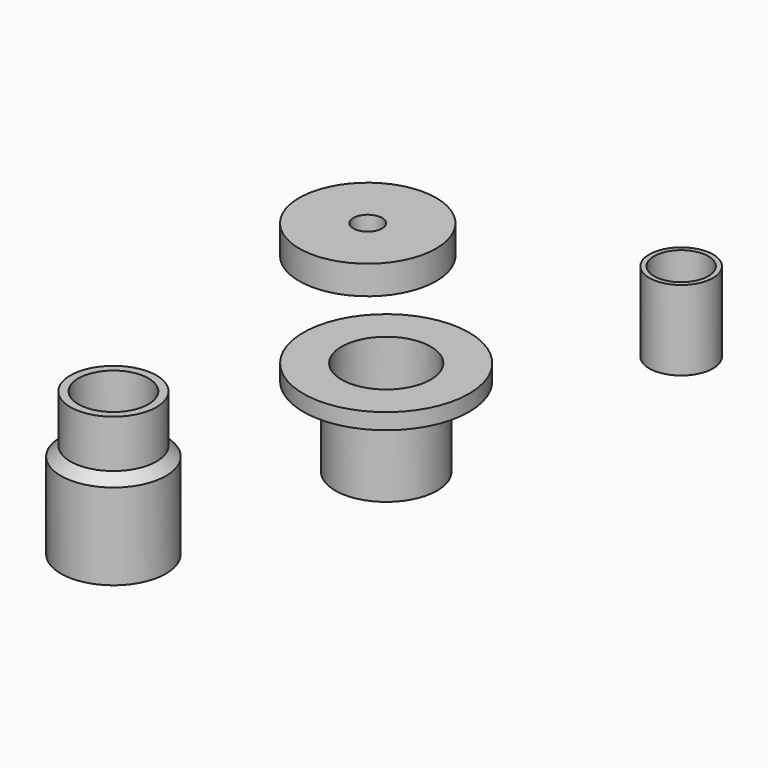
from build123d import *

# Parameters (mm, degrees)
F0_R      = 26
F0_R_2    = 14
F1_DEPTH  = 5
F2_R      = 16
F2_R_2    = 14
F3_DEPTH  = 25
F4_R      = 13.5
F4_R_2    = 11
F5_DEPTH  = 15
F6_R      = 16.5
F7_DEPTH  = 30
F8_SIZE2  = 2.99999
F8_SIZE   = 2.99999
F9_R      = 10
F9_R_2    = 2
F10_DEPTH = 25
F11_R     = 8.5
F12_DEPTH = 15
F13_R     = 3.25
F14_DEPTH = 8
F15_R     = 21.5
F15_R_2   = 4.5
F16_DEPTH = 9


# Not quite as in the source:
# - a fillet or chamfer is up to 0.001 mm smaller than in the source, because OpenCascade refuses the exact size


with BuildPart() as f1:
    # F0 (on Top) → F1 (new body)
    with BuildSketch(Plane.XY):
        Circle(F0_R)
        Circle(F0_R_2, mode=Mode.SUBTRACT)
    extrude(amount=F1_DEPTH)

    # F2 (on face) → F3 (join)
    with BuildSketch(Plane(origin=(0, 0, 0), x_dir=(1, 0, 0), z_dir=(0, 0, -1))):
        Circle(F2_R)
        Circle(F2_R_2, mode=Mode.SUBTRACT)
    extrude(amount=F3_DEPTH)


with BuildPart() as f5:
    # F4 (on Top) → F5 (new body)
    with BuildSketch(Plane.XY):
        with Locations((-48.8465763628, -45.8897389472)):
            Circle(F4_R)
        with Locations((-48.8465763628, -45.8897389472)):
            Circle(F4_R_2, mode=Mode.SUBTRACT)
    extrude(amount=-F5_DEPTH)

    # F6 (on face) → F7 (join)
    with BuildSketch(Plane(origin=(0, 0, -15), x_dir=(1, 0, 0), z_dir=(0, 0, -1))):
        with Locations((-48.8465763628, 45.8897389472)):
            Circle(F6_R)
    extrude(amount=F7_DEPTH)

    # F8 (size 3 and 3 in the source; OpenCascade refuses exactly that, so slightly less here)
    f8_edges = [f5.edges().sort_by_distance(p)[0] for p in [
        (-65.346576, -45.889739, -15),
    ]]
    chamfer(f8_edges, length=F8_SIZE, length2=F8_SIZE2)


with BuildPart() as f10:
    # F9 (on Top) → F10 (new body)
    with BuildSketch(Plane.XY):
        with Locations((48.2846722007, 55.2974492311)):
            Circle(F9_R)
        with Locations((48.2846722007, 55.2974492311)):
            Circle(F9_R_2, mode=Mode.SUBTRACT)
    extrude(amount=F10_DEPTH)

    # F11 (on face) → F12 (cut)
    with BuildSketch(Plane.XY.offset(25)):
        with Locations((48.2846722007, 55.2974492311)):
            Circle(F11_R)
    extrude(amount=-F12_DEPTH, mode=Mode.SUBTRACT)

    # F13 (on face) → F14 (cut)
    with BuildSketch(Plane.XY.offset(10)):
        with Locations((48.2846722007, 55.2974492311)):
            Circle(F13_R)
    extrude(amount=-F14_DEPTH, mode=Mode.SUBTRACT)


with BuildPart() as f16:
    # F15 (on Top) → F16 (new body)
    with BuildSketch(Plane.XY):
        with Locations((-45.1123826206, 49.1392202675)):
            Circle(F15_R)
        with Locations((-45.1123826206, 49.1392202675)):
            Circle(F15_R_2, mode=Mode.SUBTRACT)
    extrude(amount=F16_DEPTH)


solid = Compound([f1.part, f5.part, f10.part, f16.part])
